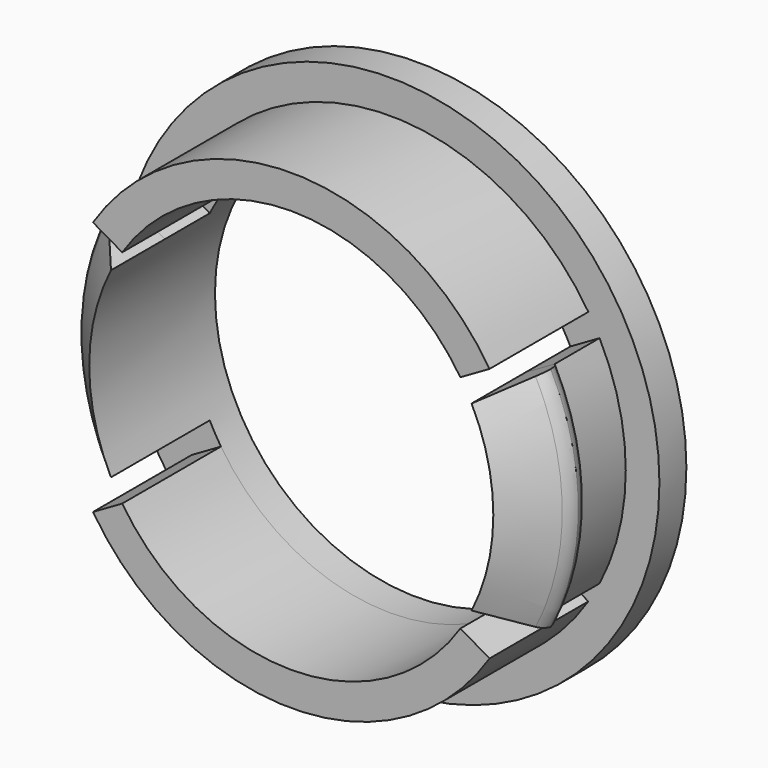
from build123d import *
from build123d import SkipClean  # not in build123d's __all__

# Parameters (mm, degrees)
F1_DEPTH     = 2.5
F2_R         = 12
F2_R_2       = 9
F3_DEPTH     = 1.5
F5_DEPTH     = 3
F6_SIZE      = 1.99999
F7_SIZE      = 0.49999
F8_T3_ANGLE  = 65.5786890643
F8_T6_ANGLE  = 65.5786890643
F8_T9_ANGLE  = 65.5786890643
F8_T12_ANGLE = 65.5786890643


# Not quite as in the source:
# - a fillet or chamfer that OpenCascade refuses, or shapes differently, is made with other operations: its cross-section is extruded or revolved along the edge and cut away or added
# - a fillet or chamfer is up to 0.001 mm smaller than in the source, because OpenCascade refuses the exact size


with BuildPart() as f1:
    # F0 (on Front) → F1 (new body)
    with BuildSketch(Plane.XZ):
        with BuildLine():
            Line((-8.0321912081, 4.060037487), (-9.3329510623, 4.811031539))
            ThreePointArc((-9.3329510623, 4.811031539), (-10.5, 0), (-9.3329510623, -4.811031539))
            Line((-9.3329510623, -4.811031539), (-8.0321912081, -4.060037487))
            ThreePointArc((-8.0321912081, -4.060037487), (-9, 0), (-8.0321912081, 4.060037487))
        make_face()
    extrude(amount=-F1_DEPTH)



with BuildPart() as f1b:
    # F0 (on Front) → F1, piece 2 (new body)
    with BuildSketch(Plane.XZ):
        with BuildLine():
            ThreePointArc((8.8329510623, 5.6770569427), (0, 10.5), (-8.8329510623, 5.6770569427))
            Line((-8.8329510623, 5.6770569427), (-7.5321912081, 4.9260628908))
            ThreePointArc((-7.5321912081, 4.9260628908), (0, 9), (7.5321912081, 4.9260628908))
            Line((7.5321912081, 4.9260628908), (8.8329510623, 5.6770569427))
        make_face()
    extrude(amount=-F1_DEPTH)


with BuildPart() as f1c:
    # F0 (on Front) → F1, piece 3 (new body)
    with BuildSketch(Plane.XZ):
        with BuildLine():
            Line((8.0321912081, -4.060037487), (9.3329510623, -4.811031539))
            ThreePointArc((9.3329510623, -4.811031539), (10.5, 0), (9.3329510623, 4.811031539))
            Line((9.3329510623, 4.811031539), (8.0321912081, 4.060037487))
            ThreePointArc((8.0321912081, 4.060037487), (9, 0), (8.0321912081, -4.060037487))
        make_face()
    extrude(amount=-F1_DEPTH)


with BuildPart() as f1d:
    # F0 (on Front) → F1, piece 4 (new body)
    with BuildSketch(Plane.XZ):
        with BuildLine():
            Line((-7.5321912081, -4.9260628908), (-8.8329510623, -5.6770569427))
            ThreePointArc((-8.8329510623, -5.6770569427), (0, -10.5), (8.8329510623, -5.6770569427))
            Line((8.8329510623, -5.6770569427), (7.5321912081, -4.9260628908))
            ThreePointArc((7.5321912081, -4.9260628908), (0, -9), (-7.5321912081, -4.9260628908))
        make_face()
    extrude(amount=-F1_DEPTH)


with BuildPart() as f1_1:
    add(f1.part, clean=False)

    add(f1b.part)  # F3 merges F1b

    add(f1c.part)  # F3 merges F1c

    add(f1d.part)  # F3 merges F1d
    # F2 (on face) → F3 (join)
    with BuildSketch(Plane(origin=(0, 2.5, 0), x_dir=(-1, 0, 0), z_dir=(0, 1, 0))):
        Circle(F2_R)
        Circle(F2_R_2, mode=Mode.SUBTRACT)
    extrude(amount=F3_DEPTH)

    # F4 (on face) → F5 (join)
    with BuildSketch(Plane.XZ):
        with BuildLine():
            ThreePointArc((-7.5321912081, 4.9260628908), (0, 9), (7.5321912081, 4.9260628908))
            Line((7.5321912081, 4.9260628908), (8.8329510623, 5.6770569427))
            ThreePointArc((8.8329510623, 5.6770569427), (0, 10.5), (-8.8329510623, 5.6770569427))
            Line((-8.8329510623, 5.6770569427), (-7.5321912081, 4.9260628908))
        make_face()
        with BuildLine():
            Line((8.0321912081, -4.060037487), (9.7664331553, -5.0613025421))
            ThreePointArc((9.7664331553, -5.0613025421), (11, 0), (9.7664331553, 5.0613025421))
            Line((9.7664331553, 5.0613025421), (8.0321912081, 4.060037487))
            ThreePointArc((8.0321912081, 4.060037487), (9, 0), (8.0321912081, -4.060037487))
        make_face()
        with BuildLine():
            Line((-8.0321912081, 4.060037487), (-9.7664331553, 5.0613025421))
            ThreePointArc((-9.7664331553, 5.0613025421), (-11, 0), (-9.7664331553, -5.0613025421))
            Line((-9.7664331553, -5.0613025421), (-8.0321912081, -4.060037487))
            ThreePointArc((-8.0321912081, -4.060037487), (-9, 0), (-8.0321912081, 4.060037487))
        make_face()
        with BuildLine():
            Line((-7.5321912081, -4.9260628908), (-8.8329510623, -5.6770569427))
            ThreePointArc((-8.8329510623, -5.6770569427), (0, -10.5), (8.8329510623, -5.6770569427))
            Line((8.8329510623, -5.6770569427), (7.5321912081, -4.9260628908))
            ThreePointArc((7.5321912081, -4.9260628908), (0, -9), (-7.5321912081, -4.9260628908))
        make_face()
    with SkipClean():  # cleaning this boolean's faces spoils the solid; the shape is the same uncleaned
        extrude(amount=F5_DEPTH)

    # F6 (size 2 in the source; OpenCascade refuses exactly that, so slightly less here)
    f6_edges = [f1_1.edges().sort_by_distance(p)[0] for p in [
        (-11, -3, 0),
        (11, -3, 0),
    ]]
    chamfer(f6_edges, length=F6_SIZE)

    # F7 (size 0.5 in the source; OpenCascade refuses exactly that, so slightly less here)
    f7_edges = [f1_1.edges().sort_by_distance(p)[0] for p in [
        (-11, 0, 0),
        (11, 0, 0),
    ]]
    chamfer(f7_edges, length=F7_SIZE)

    # F8: fillet of radius 1 on 4 edges, made by hand


with BuildPart() as f8_tool1:
    # F8_s2 → F8_t3 (revolve)
    with BuildSketch(Plane(origin=(0, 0, 0), x_dir=(0, 1, 0), z_dir=(0.5415518782, 0, 0.8406673321))):
        with BuildLine():
            ThreePointArc((-0.5857964376, 11), (-0.96847987, 10.9238795325), (-1.2929032188, 10.7071067812))
            Line((-1.2929032188, 10.7071067812), (-1.00001, 11))
            Line((-1.00001, 11), (-0.5857964376, 11))
        make_face()
    revolve(axis=Axis((0, -1.00001, 0), (0, -1, 0)), revolution_arc=F8_T3_ANGLE)


with BuildPart() as f8_tool4:
    # F8_s5 → F8_t6 (revolve)
    with BuildSketch(Plane(origin=(0, 0, 0), x_dir=(0, 1, 0), z_dir=(0.5415518782, 0, 0.8406673321))):
        with BuildLine():
            ThreePointArc((-0.9142035624, 11), (-0.53152013, 10.9238795325), (-0.2070967812, 10.7071067812))
            Line((-0.2070967812, 10.7071067812), (-0.49999, 11))
            Line((-0.49999, 11), (-0.9142035624, 11))
        make_face()
    revolve(axis=Axis((0, -0.49999, 0), (0, -1, 0)), revolution_arc=F8_T6_ANGLE)


with BuildPart() as f8_tool7:
    # F8_s8 → F8_t9 (revolve)
    with BuildSketch(Plane(origin=(0, 0, 0), x_dir=(0, 1, 0), z_dir=(-0.5415518782, 0, -0.8406673321))):
        with BuildLine():
            ThreePointArc((-0.5857964376, 11), (-0.96847987, 10.9238795325), (-1.2929032188, 10.7071067812))
            Line((-1.2929032188, 10.7071067812), (-1.00001, 11))
            Line((-1.00001, 11), (-0.5857964376, 11))
        make_face()
    revolve(axis=Axis((0, -1.00001, 0), (0, -1, 0)), revolution_arc=F8_T9_ANGLE)


with BuildPart() as f8_tool10:
    # F8_s11 → F8_t12 (revolve)
    with BuildSketch(Plane(origin=(0, 0, 0), x_dir=(0, 1, 0), z_dir=(-0.5415518782, 0, -0.8406673321))):
        with BuildLine():
            ThreePointArc((-0.9142035624, 11), (-0.53152013, 10.9238795325), (-0.2070967812, 10.7071067812))
            Line((-0.2070967812, 10.7071067812), (-0.49999, 11))
            Line((-0.49999, 11), (-0.9142035624, 11))
        make_face()
    revolve(axis=Axis((0, -0.49999, 0), (0, -1, 0)), revolution_arc=F8_T12_ANGLE)


with BuildPart() as f1_2:
    add(f1_1.part, clean=False)

    # F8_t13: cut F8_tool1, F8_tool4, F8_tool7, F8_tool10
    add([f8_tool1.part, f8_tool4.part, f8_tool7.part, f8_tool10.part], mode=Mode.SUBTRACT)


solid = f1_2.part
